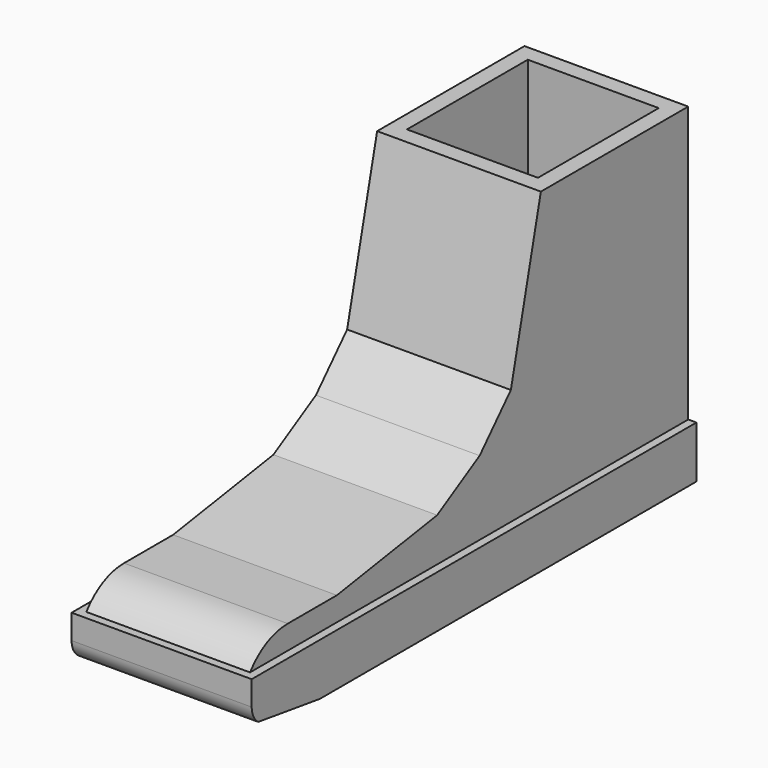
from build123d import *

# Parameters (mm, degrees)
F0_R        = 11
F0_R_2      = 8.5
F1_DEPTH    = 40
F2_T        = -4
F3_DEPTH    = 2
F5_DEPTH    = 2
F7_DEPTH    = 2
F8_T1_DEPTH = 64


# Not quite as in the source:
# - a fillet or chamfer that OpenCascade refuses, or shapes differently, is made with other operations: its cross-section is extruded or revolved along the edge and cut away or added


with BuildPart() as f1:
    # F0 (on Right) → F1 (new body)
    with BuildSketch(Plane.YZ):
        with BuildLine():
            Line((63.6921661989, -31.096493093), (63.6921661989, 38.9364992437))
            Line((63.6921661989, 38.9364992437), (18.6921661989, 38.9364992437))
            Line((18.6921661989, 38.9364992437), (9.5297960554, 0))
            Line((9.5297960554, 0), (0, -10.2558757374))
            Line((0, -10.2558757374), (-12.9771592787, -17.7787300531))
            Line((-12.9771592787, -17.7787300531), (-43.6068768529, -22.555800424))
            Line((-43.6068768529, -22.555800424), (-58.6068768529, -22.555800424))
            ThreePointArc((-58.6068768529, -22.555800424), (-65.0535615803, -24.0913867663), (-70.115709102, -28.3683520288))
            Line((-70.115709102, -28.3683520288), (-51.312591107, -31.096493093))
            Line((-51.312591107, -31.096493093), (63.6921661989, -31.096493093))
        make_face()
        with Locations((47.8400811553, 10.7847582549)):
            Circle(F0_R, mode=Mode.SUBTRACT)
        Polygon((63.6921661989, -41.0635007563), (63.6921661989, -31.096493093), (-51.312591107, -31.096493093), (-70.115709102, -28.3683520288), (-70.115709102, -38.3683520288), (-51.3078338011, -41.0635007563), align=None)
        with Locations((47.8400811553, 10.7847582549)):
            Circle(F0_R)
        with Locations((47.8400811553, 10.7847582549)):
            Circle(F0_R_2, mode=Mode.SUBTRACT)
        with Locations((47.8400811553, 10.7847582549)):
            Circle(F0_R_2)
    extrude(amount=F1_DEPTH)

    # F2
    f2_openings = [f1.faces().sort_by_distance(p)[0] for p in [
        (20, 41.192166, 38.936499),
    ]]
    offset(amount=F2_T, openings=f2_openings, kind=Kind.INTERSECTION)

    # F3 (add): a face of the model
    f3_faces = [f1.faces().sort_by_distance(p)[0] for p in [
        (20, -70.115709102, -33.3683520288),
    ]]
    extrude(f3_faces, amount=F3_DEPTH)

    # F4 (on face) → F5 (join)
    with BuildSketch(Plane.YZ.offset(40)):
        Polygon((63.6921661989, -28.3683520288), (-70.115709102, -28.3683520288), (-72.115709102, -28.3683520288), (-72.115709102, -38.3683520288), (-70.115709102, -38.3683520288), (-51.3078338011, -41.0635007563), (63.6921661989, -41.0635007563), align=None)
    extrude(amount=F5_DEPTH)

    # F6 (on face) → F7 (join)
    with BuildSketch(Plane(origin=(0, 0, 0), x_dir=(0, -1, 0), z_dir=(-1, 0, 0))):
        Polygon((72.115709102, -28.3683520288), (70.115709102, -28.3683520288), (-63.6921661989, -28.3683520288), (-63.6921661989, -41.0635007563), (51.3078338011, -41.0635007563), (70.115709102, -38.3683520288), (72.115709102, -38.3683520288), align=None)
    extrude(amount=F7_DEPTH)

    # F8: fillet of radius 5 on 1 edges, made by hand

    # F8_s2 → F8_t1 (cut)
    with BuildSketch(Plane.YZ.offset(-12)):
        with BuildLine():
            ThreePointArc((-70.115709102, -38.3683520288), (-71.587845057, -36.6044200063), (-72.115709102, -34.3683520288))
            Line((-72.115709102, -34.3683520288), (-72.115709102, -38.3683520288))
            Line((-72.115709102, -38.3683520288), (-70.115709102, -38.3683520288))
        make_face()
    extrude(amount=F8_T1_DEPTH, mode=Mode.SUBTRACT)


solid = f1.part
